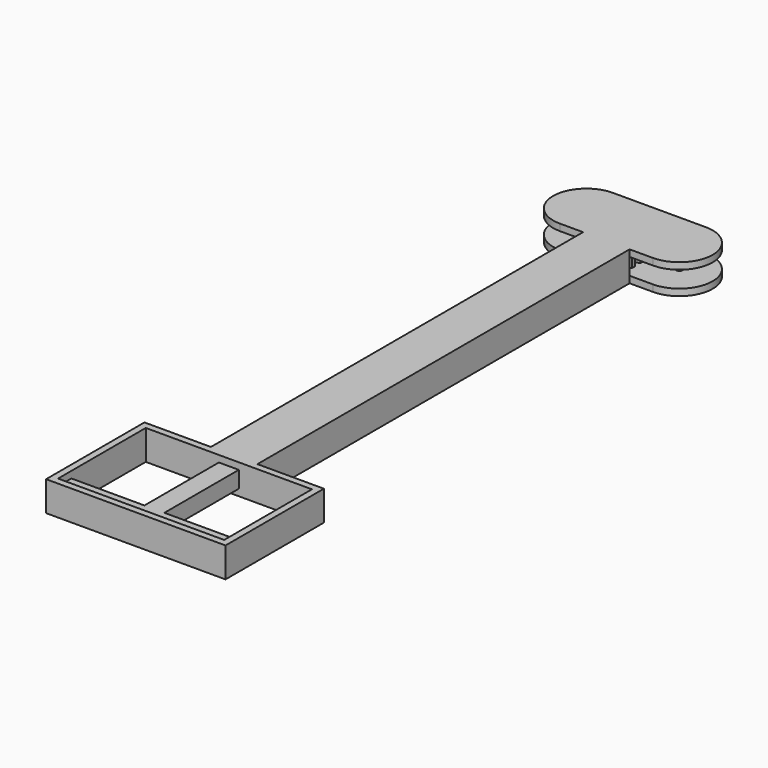
from build123d import *

# Parameters (mm, degrees)
F1_DEPTH      = 5
F3_W          = 50
F3_H          = 5
F4_DEPTH      = 5
F5_W          = 50
F5_H          = 33
F6_DEPTH      = 7
F6_DEPTH_BACK = 2
F9_DEPTH      = 5
F10_W         = 10
F10_H         = 5
F11_DEPTH     = 50
F12_R         = 1
F13_DEPTH     = 5


with BuildPart() as f1:
    # F0 (on Top) → F1 (new body)
    with BuildSketch(Plane.XY):
        Polygon((0, 13), (0, -180), (3, -180), (3, -39.0871235167), (3, -36.9128764833), (3, -35.8871235167), (3, -33.7128764833), (3, -32.6871235167), (3, -30.5128764833), (3, -29.4871235167), (3, -27.3128764833), (3, -26.2871235167), (3, -24.1128764833), (3, -23.0871235167), (3, -20.9128764833), (3, -19.8871235167), (3, -17.7128764833), (3, -16.6871235167), (3, -14.5128764833), (3, -13.4871235167), (3, -11.3128764833), (3, -10.2871235167), (3, -8.1128764833), (3, -7.0871235167), (3, -4.9128764833), (3, -3.8871235167), (3, -1.7128764833), (3, -0.6871235167), (3, 1.4871235167), (3, 2.5128764833), (3, 4.6871235167), (3, 5.7128764833), (3, 7.8871235167), (3, 8.9128764833), (3, 11.0871235167), (3, 13), align=None)
        with BuildLine():
            Line((3, -36.9128764833), (3, -39.0871235167))
            ThreePointArc((3, -39.0871235167), (4.0421988802, -38.9373096378), (5, -38.5))
            Line((5, -38.5), (5, -38))
            Line((5, -38), (5, -37.5))
            ThreePointArc((5, -37.5), (4.0421988802, -37.0626903622), (3, -36.9128764833))
        make_face()
        with BuildLine():
            ThreePointArc((5, 10.5), (4.0421988802, 10.9373096378), (3, 11.0871235167))
            Line((3, 11.0871235167), (3, 8.9128764833))
            ThreePointArc((3, 8.9128764833), (4.0421988802, 9.0626903622), (5, 9.5))
            Line((5, 9.5), (5, 10))
            Line((5, 10), (5, 10.5))
        make_face()
        with BuildLine():
            Line((3, -33.7128764833), (3, -35.8871235167))
            ThreePointArc((3, -35.8871235167), (4.0421988802, -35.7373096378), (5, -35.3))
            Line((5, -35.3), (5, -34.8))
            Line((5, -34.8), (5, -34.3))
            ThreePointArc((5, -34.3), (4.0421988802, -33.8626903622), (3, -33.7128764833))
        make_face()
        with BuildLine():
            ThreePointArc((5, 7.3), (4.0421988802, 7.7373096378), (3, 7.8871235167))
            Line((3, 7.8871235167), (3, 5.7128764833))
            ThreePointArc((3, 5.7128764833), (4.0421988802, 5.8626903622), (5, 6.3))
            Line((5, 6.3), (5, 6.8))
            Line((5, 6.8), (5, 7.3))
        make_face()
        with BuildLine():
            Line((3, -30.5128764833), (3, -32.6871235167))
            ThreePointArc((3, -32.6871235167), (4.0421988802, -32.5373096378), (5, -32.1))
            Line((5, -32.1), (5, -31.6))
            Line((5, -31.6), (5, -31.1))
            ThreePointArc((5, -31.1), (4.0421988802, -30.6626903622), (3, -30.5128764833))
        make_face()
        with BuildLine():
            ThreePointArc((5, 4.1), (4.0421988802, 4.5373096378), (3, 4.6871235167))
            Line((3, 4.6871235167), (3, 2.5128764833))
            ThreePointArc((3, 2.5128764833), (4.0421988802, 2.6626903622), (5, 3.1))
            Line((5, 3.1), (5, 3.6))
            Line((5, 3.6), (5, 4.1))
        make_face()
        with BuildLine():
            Line((3, -27.3128764833), (3, -29.4871235167))
            ThreePointArc((3, -29.4871235167), (4.0421988802, -29.3373096378), (5, -28.9))
            Line((5, -28.9), (5, -28.4))
            Line((5, -28.4), (5, -27.9))
            ThreePointArc((5, -27.9), (4.0421988802, -27.4626903622), (3, -27.3128764833))
        make_face()
        with BuildLine():
            ThreePointArc((5, 0.9), (4.0421988802, 1.3373096378), (3, 1.4871235167))
            Line((3, 1.4871235167), (3, -0.6871235167))
            ThreePointArc((3, -0.6871235167), (4.0421988802, -0.5373096378), (5, -0.1))
            Line((5, -0.1), (5, 0.4))
            Line((5, 0.4), (5, 0.9))
        make_face()
        with BuildLine():
            Line((3, -24.1128764833), (3, -26.2871235167))
            ThreePointArc((3, -26.2871235167), (4.0421988802, -26.1373096378), (5, -25.7))
            Line((5, -25.7), (5, -25.2))
            Line((5, -25.2), (5, -24.7))
            ThreePointArc((5, -24.7), (4.0421988802, -24.2626903622), (3, -24.1128764833))
        make_face()
        with BuildLine():
            ThreePointArc((5, -2.3), (4.0421988802, -1.8626903622), (3, -1.7128764833))
            Line((3, -1.7128764833), (3, -3.8871235167))
            ThreePointArc((3, -3.8871235167), (4.0421988802, -3.7373096378), (5, -3.3))
            Line((5, -3.3), (5, -2.8))
            Line((5, -2.8), (5, -2.3))
        make_face()
        with BuildLine():
            Line((3, -20.9128764833), (3, -23.0871235167))
            ThreePointArc((3, -23.0871235167), (4.0421988802, -22.9373096378), (5, -22.5))
            Line((5, -22.5), (5, -22))
            Line((5, -22), (5, -21.5))
            ThreePointArc((5, -21.5), (4.0421988802, -21.0626903622), (3, -20.9128764833))
        make_face()
        with BuildLine():
            ThreePointArc((5, -5.5), (4.0421988802, -5.0626903622), (3, -4.9128764833))
            Line((3, -4.9128764833), (3, -7.0871235167))
            ThreePointArc((3, -7.0871235167), (4.0421988802, -6.9373096378), (5, -6.5))
            Line((5, -6.5), (5, -6))
            Line((5, -6), (5, -5.5))
        make_face()
        with BuildLine():
            Line((3, -17.7128764833), (3, -19.8871235167))
            ThreePointArc((3, -19.8871235167), (4.0421988802, -19.7373096378), (5, -19.3))
            Line((5, -19.3), (5, -18.8))
            Line((5, -18.8), (5, -18.3))
            ThreePointArc((5, -18.3), (4.0421988802, -17.8626903622), (3, -17.7128764833))
        make_face()
        with BuildLine():
            ThreePointArc((5, -8.7), (4.0421988802, -8.2626903622), (3, -8.1128764833))
            Line((3, -8.1128764833), (3, -10.2871235167))
            ThreePointArc((3, -10.2871235167), (4.0421988802, -10.1373096378), (5, -9.7))
            Line((5, -9.7), (5, -9.2))
            Line((5, -9.2), (5, -8.7))
        make_face()
        with BuildLine():
            Line((3, -14.5128764833), (3, -16.6871235167))
            ThreePointArc((3, -16.6871235167), (4.0421988802, -16.5373096378), (5, -16.1))
            Line((5, -16.1), (5, -15.6))
            Line((5, -15.6), (5, -15.1))
            ThreePointArc((5, -15.1), (4.0421988802, -14.6626903622), (3, -14.5128764833))
        make_face()
        with BuildLine():
            ThreePointArc((5, -11.9), (4.0421988802, -11.4626903622), (3, -11.3128764833))
            Line((3, -11.3128764833), (3, -13.4871235167))
            ThreePointArc((3, -13.4871235167), (4.0421988802, -13.3373096378), (5, -12.9))
            Line((5, -12.9), (5, -12.4))
            Line((5, -12.4), (5, -11.9))
        make_face()
    extrude(amount=F1_DEPTH)

    # F2: F1 across face


with BuildPart() as f1_1:
    add(f1.part)
    add(f1.part.mirror(Plane(origin=(0, -83.5, 2.5), x_dir=(0, -1, 0), z_dir=(-1, 0, 0))))

    # F3 (on face) → F4 (join)
    with BuildSketch(Plane.XZ.offset(180)):
        with Locations((0, 2.5)):
            Rectangle(F3_W, F3_H)
    extrude(amount=F4_DEPTH)


with BuildPart() as f6:
    # F5 (on Top) → F6 (new body, two sides)
    with BuildSketch(Plane.XY) as f6_sk:
        with BuildLine():
            ThreePointArc((14, -10), (21.0710678119, -7.0710678119), (24, 0))
            ThreePointArc((24, 0), (21.0710678119, 7.0710678119), (14, 10))
            ThreePointArc((14, 10), (4, 0), (14, -10))
        make_face()
        with BuildLine():
            ThreePointArc((14, -10), (4, 0), (14, 10))
            Line((14, 10), (0, 10))
            Line((0, 10), (-14, 10))
            ThreePointArc((-14, 10), (-6.9289321881, 7.0710678119), (-4, 0))
            ThreePointArc((-4, 0), (-6.9289321881, -7.0710678119), (-14, -10))
            Line((-14, -10), (-7, -10))
            Line((-7, -10), (-7, -150))
            Line((-7, -150), (-27, -150))
            Line((-27, -150), (-27, -187))
            Line((-27, -187), (0, -187))
            Line((0, -187), (27, -187))
            Line((27, -187), (27, -150))
            Line((27, -150), (7, -150))
            Line((7, -150), (7, -10))
            Line((7, -10), (14, -10))
        make_face()
        with Locations((0, -168.5)):
            Rectangle(F5_W, F5_H, mode=Mode.SUBTRACT)
        with BuildLine():
            ThreePointArc((-4, 0), (-6.9289321881, 7.0710678119), (-14, 10))
            ThreePointArc((-14, 10), (-24, 0), (-14, -10))
            ThreePointArc((-14, -10), (-6.9289321881, -7.0710678119), (-4, 0))
        make_face()
    extrude(amount=F6_DEPTH)
    extrude(f6_sk.sketch, amount=-F6_DEPTH_BACK)

    # F7: cut F1
    add(f1_1.part, mode=Mode.SUBTRACT)

    # F8 (on Top) → F9 (cut)
    with BuildSketch(Plane.XY):
        with BuildLine():
            ThreePointArc((-14, 10), (-24, 0), (-14, -10))
            Line((-14, -10), (14, -10))
            ThreePointArc((14, -10), (24, 0), (14, 10))
            Line((14, 10), (-14, 10))
        make_face()
    extrude(amount=F9_DEPTH, mode=Mode.SUBTRACT)

    # F10 (on face) → F11 (cut)
    with BuildSketch(Plane(origin=(0, -10, 0), x_dir=(-1, 0, 0), z_dir=(0, 1, 0))):
        with Locations((0, 2.5)):
            Rectangle(F10_W, F10_H)
    extrude(amount=-F11_DEPTH, mode=Mode.SUBTRACT)

    # F12 (on Top) → F13 (join, through all)
    with BuildSketch(Plane.XY):
        with Locations((-14, 0)):
            Circle(F12_R)
        with Locations((14, 0)):
            Circle(F12_R)
    extrude(amount=F13_DEPTH)


solid = Compound([f1_1.part, f6.part])
